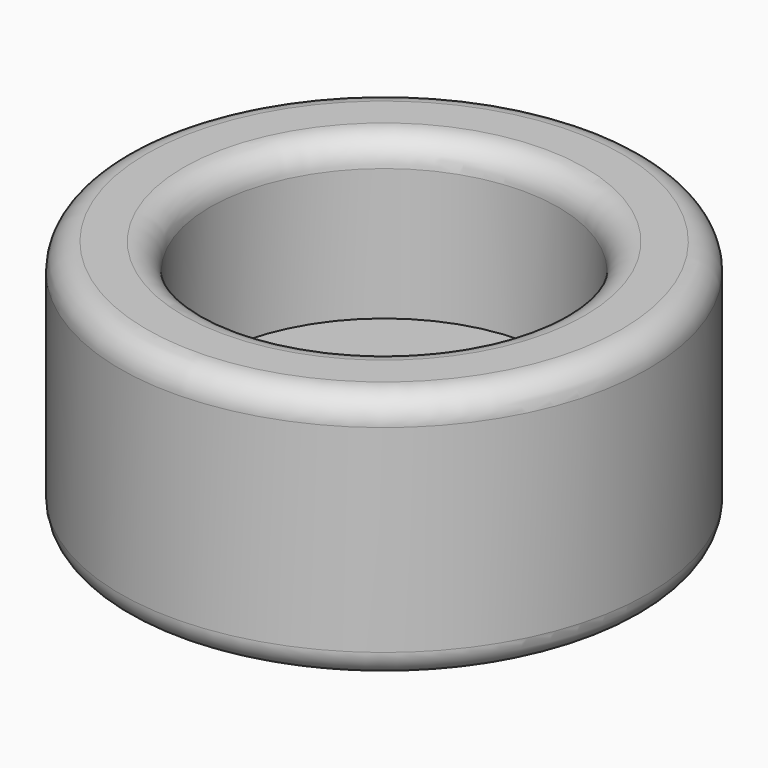
from build123d import *

# Parameters (mm, degrees)
F0_R     = 10
F1_DEPTH = 3.5
F2_R     = 10
F2_R_2   = 6.6
F3_DEPTH = 6
F4_R     = 1
F5_R     = 1
F6_R     = 0.375
F7_DEPTH = 3.501


# Not quite as in the source:
# - a feature names something its author has since deleted; it is built from what else it names


with BuildPart() as f1:
    # F0 (on Top) → F1 (new body)
    with BuildSketch(Plane.XY):
        Circle(F0_R)
    extrude(amount=-F1_DEPTH)

    # F2 (on face) → F3 (join)
    with BuildSketch(Plane.XY):
        Circle(F2_R)
        Circle(F2_R_2, mode=Mode.SUBTRACT)
    extrude(amount=F3_DEPTH)

    # F4
    f4_edges = [f1.edges().sort_by_distance(p)[0] for p in [
        (-6.6, 0, 6),
        (-10, 0, -3.5),
    ]]
    fillet(f4_edges, radius=F4_R)

    # F5
    f5_edges = [f1.edges().sort_by_distance(p)[0] for p in [
        (-10, 0, 6),
    ]]
    fillet(f5_edges, radius=F5_R)

    # F6 (on face) → F7 (cut, through all)
    with BuildSketch(Plane.XY):
        Circle(F6_R)
    extrude(amount=-F7_DEPTH, mode=Mode.SUBTRACT)


solid = f1.part
